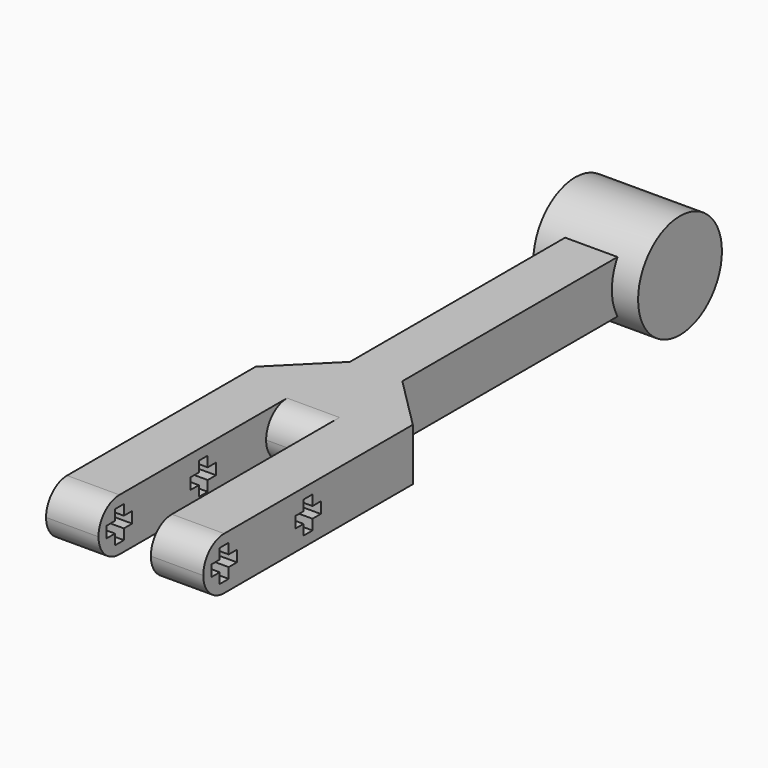
from build123d import *

# Parameters (mm, degrees)
F1_DEPTH     = 7.9375
F2_R         = 3.96874
F3_W         = 1.56845
F3_H         = 1.6891
F3_W_2       = 1.6891
F3_H_2       = 1.56845
F4_DEPTH     = 130
F5_SIZE      = 7.93749
F6_W         = 15.875
F6_H         = 15.875
F7_DEPTH     = 15.875
F8_T1_DEPTH  = 55.5625
F8_T6_DEPTH  = 55.5625
F8_T12_DEPTH = 55.5625
F8_T18_DEPTH = 55.5625
F8_T25_DEPTH = 55.5625
F8_T31_DEPTH = 55.5625
F8_T37_DEPTH = 55.5625
F8_T43_DEPTH = 55.5625
F8_T49_DEPTH = 55.5625
F8_T56_DEPTH = 55.5625
F8_T62_DEPTH = 55.5625


# Not quite as in the source:
# - a fillet or chamfer that OpenCascade refuses, or shapes differently, is made with other operations: its cross-section is extruded or revolved along the edge and cut away or added
# - a fillet or chamfer is up to 0.001 mm smaller than in the source, because OpenCascade refuses the exact size
# - an extrude ends at something that could not be found from the text; its depth is read off the source's solid


with BuildPart() as f1:
    # F0 (on Top) → F1 (new body)
    with BuildSketch(Plane.XY):
        Polygon((0, 39.6875), (0, 0), (7.9375, 0), (7.9375, 31.75), (15.875, 31.75), (15.875, 0), (23.8125, 0), (23.8125, 39.6875), (15.875, 39.6875), (15.875, 87.3125), (7.9375, 87.3125), (7.9375, 39.6875), align=None)
    extrude(amount=F1_DEPTH)

    # F2 (radius 3.96875 in the source; OpenCascade refuses exactly that, so slightly less here)
    f2_edges = [f1.edges().sort_by_distance(p)[0] for p in [
        (3.96875, 0, 0),
        (3.96875, 0, 7.9375),
        (19.84375, 0, 7.9375),
        (19.84375, 0, 0),
        (11.90625, 31.75, 7.9375),
        (11.90625, 31.75, 0),
    ]]
    fillet(f2_edges, radius=F2_R)

    # F3 (on face) → F4 (cut, through all)
    with BuildSketch(Plane(origin=(0, 0, 0), x_dir=(0, -1, 0), z_dir=(-1, 0, 0))):
        with Locations((-2.339975, 3.96875)):
            Rectangle(F3_W, F3_H)
        with Locations((-3.96875, 2.339975)):
            Rectangle(F3_W_2, F3_H_2)
        with Locations((-3.96875, 3.96875)):
            Rectangle(F3_W_2, F3_H)
        with Locations((-5.597525, 3.96875)):
            Rectangle(F3_W, F3_H)
        with Locations((-3.96875, 5.597525)):
            Rectangle(F3_W_2, F3_H_2)
        with Locations((-19.84375, 2.339975)):
            Rectangle(F3_W_2, F3_H_2)
        with Locations((-21.472525, 3.96875)):
            Rectangle(F3_W, F3_H)
        with Locations((-19.84375, 3.96875)):
            Rectangle(F3_W_2, F3_H)
        with Locations((-18.214975, 3.96875)):
            Rectangle(F3_W, F3_H)
        with Locations((-19.84375, 5.597525)):
            Rectangle(F3_W_2, F3_H_2)
    extrude(amount=-F4_DEPTH, mode=Mode.SUBTRACT)

    # F5 (size 7.9375 in the source; OpenCascade refuses exactly that, so slightly less here)
    f5_edges = [f1.edges().sort_by_distance(p)[0] for p in [
        (7.9375, 39.6875, 3.96875),
        (15.875, 39.6875, 3.96875),
    ]]
    chamfer(f5_edges, length=F5_SIZE)

    # F6 (on face) → F7 (join)
    with BuildSketch(Plane(origin=(0, 87.3125, 0), x_dir=(-1, 0, 0), z_dir=(0, 1, 0))):
        with Locations((-11.90625, 3.96875)):
            Rectangle(F6_W, F6_H)
    extrude(amount=F7_DEPTH)

    # F8: fillet of radius 7.9375 on 4 edges, made by hand

    # F8_s2 → F8_t1 (cut)
    with BuildSketch(Plane.YZ.offset(-15.875)):
        with BuildLine():
            ThreePointArc((95.25, -3.96875), (100.8626600757, -1.6439100757), (103.1875, 3.96875))
            Line((103.1875, 3.96875), (103.1875, -3.96875))
            Line((103.1875, -3.96875), (95.25, -3.96875))
        make_face()
        with BuildLine():
            ThreePointArc((95.25, 11.90625), (100.8626600757, 9.5814100757), (103.1875, 3.96875))
            Line((103.1875, 3.96875), (103.1875, 11.90625))
            Line((103.1875, 11.90625), (95.25, 11.90625))
        make_face()
    extrude(amount=F8_T1_DEPTH, mode=Mode.SUBTRACT)


with BuildPart() as f8_tool4:
    # F8_s5 → F8_t6 (new body)
    with BuildSketch(Plane.YZ.offset(39.6875)):
        with BuildLine():
            ThreePointArc((95.25, -3.96875), (89.6373399243, -1.6439100757), (87.3125, 3.96875))
            Line((87.3125, 3.96875), (87.3125, -3.96875))
            Line((87.3125, -3.96875), (95.25, -3.96875))
        make_face()
    extrude(amount=-F8_T6_DEPTH)

    split(bisect_by=Plane.XY, keep=Keep.BOTTOM)

    split(bisect_by=Plane.YZ.offset(15.875), keep=Keep.TOP)


with BuildPart() as f1_1:
    add(f1.part)

    # F8_t3: cut F8_tool4
    add(f8_tool4.part, mode=Mode.SUBTRACT)


with BuildPart() as f8_tool10:
    # F8_s11 → F8_t12 (new body)
    with BuildSketch(Plane.YZ.offset(39.6875)):
        with BuildLine():
            ThreePointArc((95.25, -3.96875), (89.6373399243, -1.6439100757), (87.3125, 3.96875))
            Line((87.3125, 3.96875), (87.3125, -3.96875))
            Line((87.3125, -3.96875), (95.25, -3.96875))
        make_face()
    extrude(amount=-F8_T12_DEPTH)

    split(bisect_by=Plane.XY, keep=Keep.TOP)

    split(bisect_by=Plane.YZ.offset(15.875), keep=Keep.TOP)


with BuildPart() as f1_2:
    add(f1_1.part)

    # F8_t9: cut F8_tool10
    add(f8_tool10.part, mode=Mode.SUBTRACT)


with BuildPart() as f8_tool16:
    # F8_s17 → F8_t18 (new body)
    with BuildSketch(Plane.YZ.offset(39.6875)):
        with BuildLine():
            ThreePointArc((95.25, -3.96875), (89.6373399243, -1.6439100757), (87.3125, 3.96875))
            Line((87.3125, 3.96875), (87.3125, -3.96875))
            Line((87.3125, -3.96875), (95.25, -3.96875))
        make_face()
    extrude(amount=-F8_T18_DEPTH)

    split(bisect_by=Plane.XY, keep=Keep.BOTTOM)

    split(bisect_by=Plane.YZ.offset(7.9375), keep=Keep.TOP)

    split(bisect_by=Plane.YZ.offset(15.875), keep=Keep.BOTTOM)


with BuildPart() as f1_3:
    add(f1_2.part)

    # F8_t15: cut F8_tool16
    add(f8_tool16.part, mode=Mode.SUBTRACT)


with BuildPart() as f8_tool23:
    # F8_s24 → F8_t25 (new body)
    with BuildSketch(Plane.YZ.offset(39.6875)):
        with BuildLine():
            ThreePointArc((95.25, -3.96875), (89.6373399243, -1.6439100757), (87.3125, 3.96875))
            Line((87.3125, 3.96875), (87.3125, -3.96875))
            Line((87.3125, -3.96875), (95.25, -3.96875))
        make_face()
    extrude(amount=-F8_T25_DEPTH)

    split(bisect_by=Plane.XY, keep=Keep.BOTTOM)

    split(bisect_by=Plane.YZ.offset(7.9375), keep=Keep.BOTTOM)


with BuildPart() as f1_4:
    add(f1_3.part)

    # F8_t22: cut F8_tool23
    add(f8_tool23.part, mode=Mode.SUBTRACT)


with BuildPart() as f8_tool29:
    # F8_s30 → F8_t31 (new body)
    with BuildSketch(Plane.YZ.offset(39.6875)):
        with BuildLine():
            ThreePointArc((95.25, -3.96875), (89.6373399243, -1.6439100757), (87.3125, 3.96875))
            Line((87.3125, 3.96875), (87.3125, -3.96875))
            Line((87.3125, -3.96875), (95.25, -3.96875))
        make_face()
    extrude(amount=-F8_T31_DEPTH)

    split(bisect_by=Plane.XY, keep=Keep.TOP)

    split(bisect_by=Plane.YZ.offset(7.9375), keep=Keep.BOTTOM)


with BuildPart() as f1_5:
    add(f1_4.part)

    # F8_t28: cut F8_tool29
    add(f8_tool29.part, mode=Mode.SUBTRACT)


with BuildPart() as f8_tool35:
    # F8_s36 → F8_t37 (new body)
    with BuildSketch(Plane.YZ.offset(-15.875)):
        with BuildLine():
            ThreePointArc((95.25, 11.90625), (89.6373399243, 9.5814100757), (87.3125, 3.96875))
            Line((87.3125, 3.96875), (87.3125, 11.90625))
            Line((87.3125, 11.90625), (95.25, 11.90625))
        make_face()
    extrude(amount=F8_T37_DEPTH)

    split(bisect_by=Plane.YZ.offset(7.9375), keep=Keep.BOTTOM)

    split(bisect_by=Plane.XY.offset(7.9375), keep=Keep.TOP)


with BuildPart() as f1_6:
    add(f1_5.part)

    # F8_t34: cut F8_tool35
    add(f8_tool35.part, mode=Mode.SUBTRACT)


with BuildPart() as f8_tool41:
    # F8_s42 → F8_t43 (new body)
    with BuildSketch(Plane.YZ.offset(-15.875)):
        with BuildLine():
            ThreePointArc((95.25, 11.90625), (89.6373399243, 9.5814100757), (87.3125, 3.96875))
            Line((87.3125, 3.96875), (87.3125, 11.90625))
            Line((87.3125, 11.90625), (95.25, 11.90625))
        make_face()
    extrude(amount=F8_T43_DEPTH)

    split(bisect_by=Plane.YZ.offset(7.9375), keep=Keep.BOTTOM)

    split(bisect_by=Plane.XY.offset(7.9375), keep=Keep.BOTTOM)


with BuildPart() as f1_7:
    add(f1_6.part)

    # F8_t40: cut F8_tool41
    add(f8_tool41.part, mode=Mode.SUBTRACT)


with BuildPart() as f8_tool47:
    # F8_s48 → F8_t49 (new body)
    with BuildSketch(Plane.YZ.offset(-15.875)):
        with BuildLine():
            ThreePointArc((95.25, 11.90625), (89.6373399243, 9.5814100757), (87.3125, 3.96875))
            Line((87.3125, 3.96875), (87.3125, 11.90625))
            Line((87.3125, 11.90625), (95.25, 11.90625))
        make_face()
    extrude(amount=F8_T49_DEPTH)

    split(bisect_by=Plane.YZ.offset(7.9375), keep=Keep.TOP)

    split(bisect_by=Plane.XY.offset(7.9375), keep=Keep.TOP)

    split(bisect_by=Plane.YZ.offset(15.875), keep=Keep.BOTTOM)


with BuildPart() as f1_8:
    add(f1_7.part)

    # F8_t46: cut F8_tool47
    add(f8_tool47.part, mode=Mode.SUBTRACT)


with BuildPart() as f8_tool54:
    # F8_s55 → F8_t56 (new body)
    with BuildSketch(Plane.YZ.offset(-15.875)):
        with BuildLine():
            ThreePointArc((95.25, 11.90625), (89.6373399243, 9.5814100757), (87.3125, 3.96875))
            Line((87.3125, 3.96875), (87.3125, 11.90625))
            Line((87.3125, 11.90625), (95.25, 11.90625))
        make_face()
    extrude(amount=F8_T56_DEPTH)

    split(bisect_by=Plane.XY.offset(7.9375), keep=Keep.TOP)

    split(bisect_by=Plane.YZ.offset(15.875), keep=Keep.TOP)


with BuildPart() as f1_9:
    add(f1_8.part)

    # F8_t53: cut F8_tool54
    add(f8_tool54.part, mode=Mode.SUBTRACT)


with BuildPart() as f8_tool60:
    # F8_s61 → F8_t62 (new body)
    with BuildSketch(Plane.YZ.offset(-15.875)):
        with BuildLine():
            ThreePointArc((95.25, 11.90625), (89.6373399243, 9.5814100757), (87.3125, 3.96875))
            Line((87.3125, 3.96875), (87.3125, 11.90625))
            Line((87.3125, 11.90625), (95.25, 11.90625))
        make_face()
    extrude(amount=F8_T62_DEPTH)

    split(bisect_by=Plane.XY.offset(7.9375), keep=Keep.BOTTOM)

    split(bisect_by=Plane.YZ.offset(15.875), keep=Keep.TOP)


with BuildPart() as f1_10:
    add(f1_9.part)

    # F8_t59: cut F8_tool60
    add(f8_tool60.part, mode=Mode.SUBTRACT)


solid = f1_10.part
